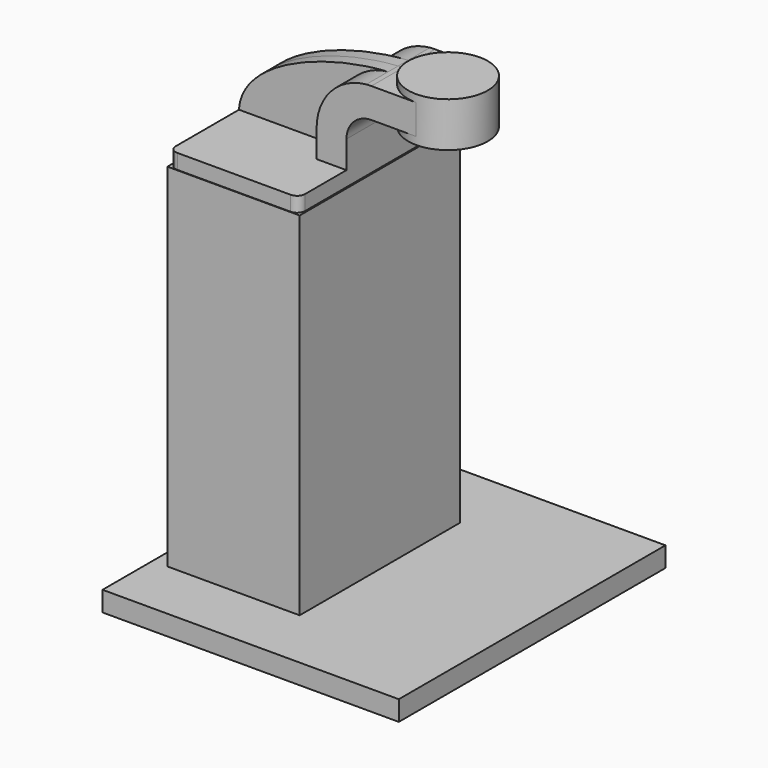
from build123d import *

# Parameters (mm, degrees)
F1_DEPTH  = 63.5
F0_W      = 25.4
F0_H      = 19.05
F2_DEPTH  = 25.4
F3_DEPTH  = 7.9375
F5_R      = 5.08
F6_W      = 84.3743681908
F6_H      = 127.7539134026
F7_DEPTH  = 229.7079414129
F8_W      = 212.6137167215
F8_H      = 12.7539038658
F9_DEPTH  = 51.7011582851
F10_DEPTH = 85.5997037143


# Not quite as in the source:
# - the program builds the solid bodies; features that only make, move or delete a surface that nothing else refers to are left out


with BuildPart() as f1:
    # F0 (on Front) → F1 (new body, symmetric)
    with BuildSketch(Plane.XZ):
        Polygon((22.225, 9.525), (-41.275, 9.525), (-41.275, -9.525), (41.275, -9.525), (41.275, 9.525), align=None)
    extrude(amount=F1_DEPTH, both=True)

    # F0 (on Front) → F2 (join, symmetric)
    with BuildSketch(Plane.XZ):
        with BuildLine():
            Line((22.225, 27.0002), (22.225, 9.525))
            Line((22.225, 9.525), (41.275, 9.525))
            Line((41.275, 9.525), (41.275, 27.0002))
            ThreePointArc((41.275, 27.0002), (45.9246798487, 38.2255201513), (57.15, 42.8752))
            Line((57.15, 42.8752), (60.325, 42.8752))
            Line((60.325, 42.8752), (60.325, 61.9252))
            Line((60.325, 61.9252), (57.15, 61.9252))
            add(Edge.make_bspline(
                [(53.8854342407, 61.7722898912), (54.9842067368, 61.8365871986), (56.0728453275, 61.8876096574), (57.15, 61.9252)],
                knots=[108.5245810491, 108.5245810491, 108.5245810491, 108.5245810491, 111.5045361635, 111.5045361635, 111.5045361635, 111.5045361635], degree=3))
            ThreePointArc((53.8854342407, 61.7722898912), (31.3258777096, 50.5133948686), (22.225, 27.0002))
        make_face()
        with Locations((73.025, 52.4002)):
            Rectangle(F0_W, F0_H)
    extrude(amount=F2_DEPTH, both=True)

    # F0 (on Front) → F3 (join, symmetric)
    with BuildSketch(Plane.XZ):
        with BuildLine():
            add(Edge.make_bspline(
                [(-41.275, 9.525), (-39.5856284224, 39.4828766469), (13.870125209, 59.4306981306), (53.8854342407, 61.7722898912)],
                knots=[0, 0, 0, 0, 108.5245810491, 108.5245810491, 108.5245810491, 108.5245810491], degree=3))
            Line((-41.275, 9.525), (22.225, 9.525))
            Line((22.225, 9.525), (22.225, 27.0002))
            ThreePointArc((22.225, 27.0002), (31.3258777096, 50.5133948686), (53.8854342407, 61.7722898912))
        make_face()
    extrude(amount=F3_DEPTH, both=True)

    # F0 (on Front) → F4 (revolve)
    with BuildSketch(Plane.XZ):
        Polygon((85.725, 66.675), (85.725, 61.9252), (85.725, 42.8752), (85.725, 38.1), (111.125, 38.1), (111.125, 66.675), align=None)
    revolve(axis=Axis((85.725, 0, 52.3875), (0, 0, 1)))

    # F5
    f5_edges = [f1.edges().sort_by_distance(p)[0] for p in [
        (41.275, -63.5, 0),
        (-41.275, -63.5, 0),
        (41.275, 63.5, 0),
        (-41.275, 63.5, 0),
    ]]
    fillet(f5_edges, radius=F5_R)

    # F6 (on Top) → F7 (join)
    with BuildSketch(Plane.XY):
        Rectangle(F6_W, F6_H)
    extrude(amount=-F7_DEPTH)

    # F8 (on Right) → F9 (join, symmetric)
    with BuildSketch(Plane.YZ):
        with Locations((2.6118680835, -230.9240400791)):
            Rectangle(F8_W, F8_H)
    extrude(amount=F9_DEPTH, both=True)

    # F10 (add): a face of the model
    f10_faces = [f1.faces().sort_by_distance(p)[0] for p in [
        (51.7011582851, 2.6118680835, -230.9240400791),
    ]]
    extrude(f10_faces, amount=F10_DEPTH)


solid = f1.part
